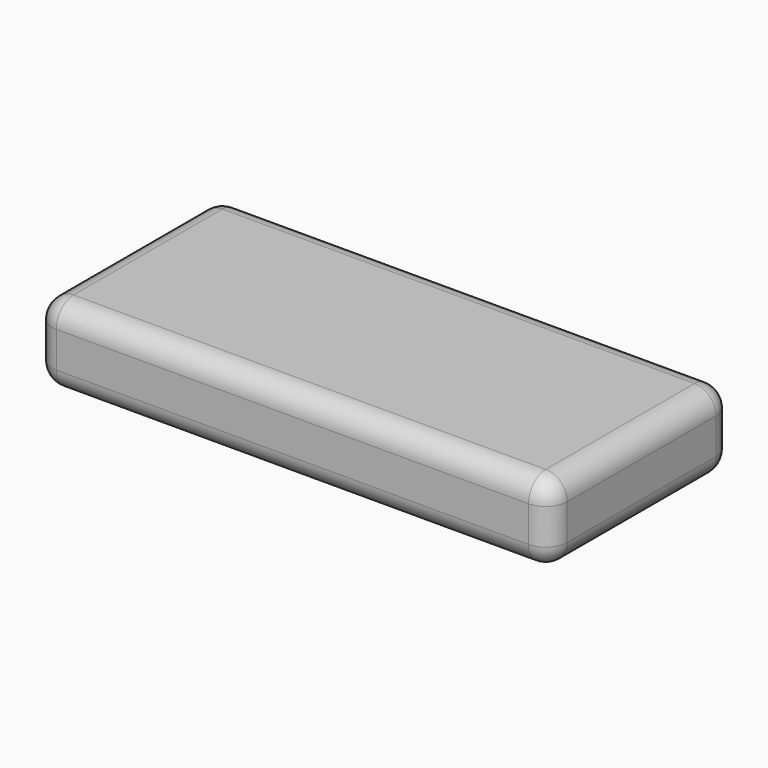
from build123d import *

# Parameters (mm, degrees)
F0_W     = 45.72
F0_H     = 6.985
F1_DEPTH = 10.16
F2_R     = 1.905
F6_ANGLE = 180
F3_W     = 12.446
F3_H     = 2.286
F7_DEPTH = 5.207
F4_W     = 7.62
F4_H     = 1.778
F8_DEPTH = 7.8105


# Not quite as in the source:
# - a length typed as a fraction of an inch, garbled in the dataset ("3 / 203.2 mm" for 3/8 in), is restored


with BuildPart() as f1:
    # F0 (on Front) → F1 (new body)
    with BuildSketch(Plane.XZ):
        Rectangle(F0_W, F0_H)
    extrude(amount=-F1_DEPTH)

    # F2
    f2_edges = [f1.edges().sort_by_distance(p)[0] for p in [
        (0, 10.16, 3.4925),
        (22.86, 5.08, 3.4925),
        (22.86, 10.16, 0),
        (22.86, 5.08, -3.4925),
        (-22.86, 10.16, 0),
        (-22.86, 5.08, -3.4925),
        (-22.86, 5.08, 3.4925),
        (0, 10.16, -3.4925),
    ]]
    fillet(f2_edges, radius=F2_R)

    # F5 (on face) → F6 (revolve, cut)
    with BuildSketch(Plane.XZ):
        Polygon((13.97, -1.5621), (18.542, -0.5461), (18.542, 0.5969), (20.32, 0.5969), (20.32, 2.3749), (12.446, 2.3749), (12.446, -3.0861), (13.97, -3.0861), align=None)
    revolve(axis=Axis((12.446, 0, -0.3556), (0, 0, 1)), revolution_arc=F6_ANGLE, mode=Mode.SUBTRACT)

    # F3 (on face) → F7 (cut)
    with BuildSketch(Plane.XZ):
        with Locations((-14.097, 0)):
            Rectangle(F3_W, F3_H)
    extrude(amount=-F7_DEPTH, mode=Mode.SUBTRACT)

    # F4 (on face) → F8 (cut)
    with BuildSketch(Plane.XZ):
        with Locations((-1.27, 0)):
            Rectangle(F4_W, F4_H)
    extrude(amount=-F8_DEPTH, mode=Mode.SUBTRACT)

    # F9: F1 across face


with BuildPart() as f1_1:
    add(f1.part)
    add(f1.part.mirror(Plane(origin=(-1.1723055417, 0, -0.108173269), x_dir=(1, 0, 0), z_dir=(0, -1, 0))))


solid = f1_1.part
